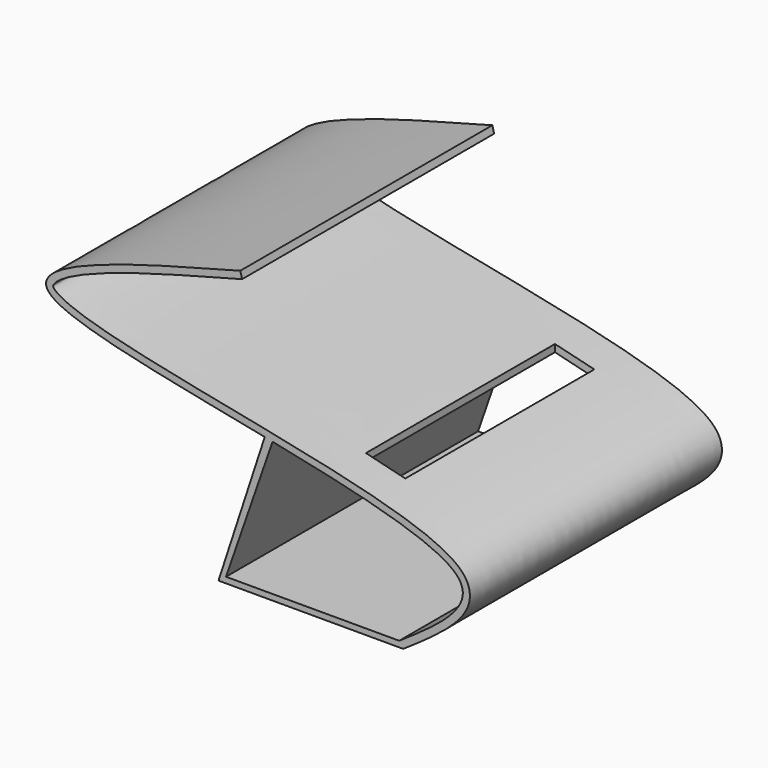
from build123d import *

# Parameters (mm, degrees)
F1_DEPTH = 101.6
F2_W     = 12.7
F2_H     = 76.2
F3_DEPTH = 25.4


# Not quite as in the source:
# - the dataset's text gives a spline's control points without its knots; the knots are read off the source's solid


with BuildPart() as f1:
    # F0 (on Front) → F1 (new body)
    with BuildSketch(Plane.XZ):
        with BuildLine():
            Line((-29.7689282068, 44.5325319117), (-30.3504820913, 46.7433221638))
            add(Edge.make_bspline(
                [(-30.3504820913, 46.7433221638), (-65.4792465579, 37.5026131401), (-126.9359011048, 21.3362870293), (-53.1419871092, 8.2662800236), (-22.4746837858, 2.097254196)],
                knots=[0, 0, 0, 0, 0.3218240885, 0.5630209925, 0.5630209925, 0.5630209925, 0.5630209925], degree=3))
            Line((-22.4746837858, 2.097254196), (-37.3928770423, -43.5353918503))
            Line((-37.3928770423, -43.5353918503), (22.1730041869, -43.5353918503))
            add(Edge.make_bspline(
                [(-29.7689282068, 44.5325319117), (-33.1800274027, 43.6352337688), (-39.998341745, 41.8416533056), (-49.9706338774, 39.160194504), (-59.4424633937, 36.494232515), (-68.1657748481, 33.8517051844), (-74.6008981086, 31.6777905715), (-79.1164276054, 29.964768348), (-82.151587871, 28.6972263494), (-84.7980091363, 27.4533776691), (-87.014479639, 26.2447291833), (-88.7545811685, 25.0939135409), (-89.7626771944, 24.2215801126), (-90.2841053939, 23.6282062584), (-90.5358874781, 23.2570539545), (-90.6641591658, 22.9815588437), (-90.7052678374, 22.8114230075), (-90.7077430294, 22.7177398154), (-90.6937600848, 22.6247603025), (-90.6298038157, 22.4558990126), (-90.4551017544, 22.1819113739), (-90.1249027626, 21.8158928441), (-89.4405221889, 21.2325249423), (-88.1101599753, 20.3801381613), (-85.8552568912, 19.2917040843), (-83.0189760989, 18.1754171095), (-79.6647858948, 17.0486594734), (-74.5739362939, 15.5404642857), (-67.1748533538, 13.6508299997), (-57.005464278, 11.375565199), (-45.8940580008, 9.0822116846), (-34.182858287, 6.7579039526), (-22.2103642832, 4.3884059772), (-10.3126752643, 1.958720781), (1.1765238168, -0.5470106193), (11.9267687798, -3.1459247063), (21.613631095, -5.858469164), (28.5386885644, -8.2360797133), (33.2491780436, -10.2364505596), (36.3379175047, -11.8010225513), (38.5220292101, -13.1806613757), (40.0238851524, -14.3575877569), (41.025282446, -15.2912304345), (41.885875849, -16.2836675268), (42.5927779455, -17.3330279302), (43.1368949429, -18.4399632147), (43.6294941624, -19.9771565027), (43.7845017363, -21.9589304675), (43.3084967659, -24.2408004362), (42.3375941541, -26.37071833), (40.9843153221, -28.3893021336), (39.3128239767, -30.3414661856), (36.7194836379, -32.8955374316), (32.8918930664, -36.0426029128), (27.6751327821, -39.80032588), (24.0015427317, -42.2940363483), (22.1730041869, -43.5353918503)],
                knots=[0, 0, 0, 0, 0.03125, 0.0625, 0.09375, 0.125, 0.15625, 0.171875, 0.1875, 0.203125, 0.21875, 0.234375, 0.25, 0.2578125, 0.265625, 0.2734375, 0.28125, 0.2890625, 0.296875, 0.3046875, 0.3125, 0.3203125, 0.328125, 0.34375, 0.359375, 0.375, 0.390625, 0.40625, 0.4375, 0.46875, 0.5, 0.53125, 0.5625, 0.59375, 0.625, 0.65625, 0.6875, 0.71875, 0.734375, 0.75, 0.765625, 0.7734375, 0.78125, 0.7890625, 0.796875, 0.8046875, 0.8125, 0.828125, 0.84375, 0.859375, 0.875, 0.890625, 0.90625, 0.9375, 0.96875, 1, 1, 1, 1], degree=3))
        make_face()
        with BuildLine():
            Line((-34.9644646049, -41.644051671), (-19.9553178139, 1.588615424))
            add(Edge.make_bspline(
                [(-19.9553178139, 1.588615424), (6.871230209, -3.8485104187), (58.8789404783, -15.8535074244), (33.6967682905, -32.9491426714), (20.8890140057, -41.644051671)],
                knots=[0.5696328726, 0.5696328726, 0.5696328726, 0.5696328726, 0.7811135442, 1, 1, 1, 1], degree=3))
            Line((20.8890140057, -41.644051671), (-34.9644646049, -41.644051671))
        make_face(mode=Mode.SUBTRACT)
    extrude(amount=F1_DEPTH)

    # F2 (on Top) → F3 (cut)
    with BuildSketch(Plane.XY):
        with Locations((6.35, -50.8)):
            Rectangle(F2_W, F2_H)
    extrude(amount=-F3_DEPTH, mode=Mode.SUBTRACT)


solid = f1.part
